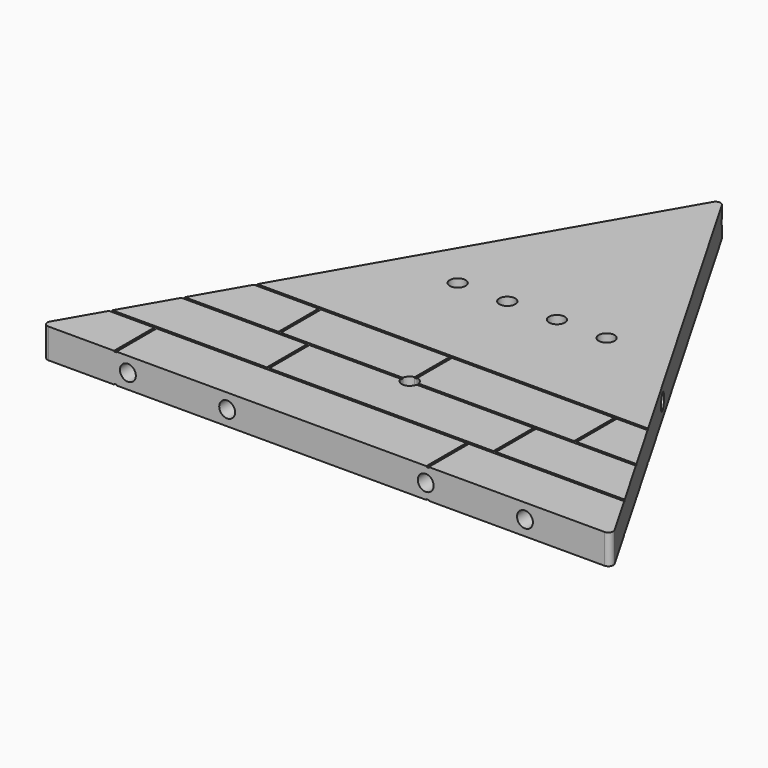
from build123d import *

# Parameters (mm, degrees)
F3_DEPTH       = 6
F4_W           = 32.6863850343
F4_H           = 10.1006624426
F4_W_2         = 25.8918322674
F5_DEPTH       = 0.15
F6_W           = 25.8918322674
F6_H           = 10.1006624426
F6_W_2         = 45.1567518413
F6_W_3         = 32.6863850343
F7_DEPTH       = 0.15
F8_R           = 1.6
F9_DEPTH       = 5
F11_R          = 1.05
F12_DEPTH      = 5
F12_DEPTH_BACK = 0.501
F13_R          = 1.6
F14_DEPTH      = 5
F15_R          = 1.6
F16_DEPTH      = 5
F17_R          = 1.6
F18_DEPTH      = 5


with BuildPart() as f3:
    # F2 (on Top) → F3 (new body)
    with BuildSketch(Plane.XY):
        with BuildLine():
            ThreePointArc((0.8660254038, 98.5), (0, 99), (-0.8660254038, 98.5))
            Line((-0.8660254038, 98.5), (-56.8690015152, 1.5))
            ThreePointArc((-56.8690015152, 1.5), (-56.8690015152, 0.5), (-56.0029761114, 0))
            Line((-56.0029761114, 0), (56.0029761114, 0))
            ThreePointArc((56.0029761114, 0), (56.8690015152, 0.5), (56.8690015152, 1.5))
            Line((56.8690015152, 1.5), (0.8660254038, 98.5))
        make_face()
    extrude(amount=F3_DEPTH)

    # F4 (on face) → F5 (cut)
    with BuildSketch(Plane.XY.offset(6)):
        Polygon((39.6628161091, 31.3019873277), (39.3741409745, 31.8019873277), (0, 31.8019873277), (0, 20.7013248852), (25.1688986466, 20.7013248852), (25.1688986466, 10.6006624426), (0, 10.6006624426), (0, 10.1006624426), (20.1229155064, 10.1006624426), (20.1229155064, 0), (20.6229155064, 0), (20.6229155064, 10.1006624426), (51.9034067387, 10.1006624426), (51.6147316042, 10.6006624426), (25.6688986466, 10.6006624426), (25.6688986466, 20.7013248852), (45.7831114239, 20.7013248852), (45.4944362893, 21.2013248852), (33.4497465572, 21.2013248852), (33.4497465572, 31.3019873277), align=None)
        with Locations((16.60655404, 26.2516561065)):
            Rectangle(F4_W, F4_H, mode=Mode.SUBTRACT)
        Polygon((0, 20.7013248852), (0, 31.8019873277), (-39.3741409745, 31.8019873277), (-39.6628161091, 31.3019873277), (-26.6284707446, 31.3019873277), (-26.6284707446, 21.2013248852), (-45.4944362893, 21.2013248852), (-45.7831114239, 20.7013248852), (-20.4878531947, 20.7013248852), (-20.4878531947, 10.6006624426), (-51.6147316042, 10.6006624426), (-51.9034067387, 10.1006624426), (-42.7899323404, 10.1006624426), (-42.7899323404, 0), (-42.2899323404, 0), (-42.2899323404, 10.1006624426), (0, 10.1006624426), (0, 10.6006624426), (-19.9878531947, 10.6006624426), (-19.9878531947, 20.7013248852), align=None)
        with Locations((-13.1825546109, 26.2516561065)):
            Rectangle(F4_W_2, F4_H, mode=Mode.SUBTRACT)
    extrude(amount=-F5_DEPTH, mode=Mode.SUBTRACT)

    # F6 (on face) → F7 (cut)
    with BuildSketch(Plane.XY):
        Polygon((-51.9034067387, 10.1006624426), (-42.7899323404, 10.1006624426), (-42.7899323404, 0), (-42.2899323404, 0), (-42.2899323404, 10.1006624426), (20.1229155064, 10.1006624426), (20.1229155064, 0), (20.6229155064, 0), (20.6229155064, 10.1006624426), (51.9034067387, 10.1006624426), (51.6147316042, 10.6006624426), (25.6688986466, 10.6006624426), (25.6688986466, 20.7013248852), (45.7831114239, 20.7013248852), (45.4944362893, 21.2013248852), (33.4497465572, 21.2013248852), (33.4497465572, 31.3019873277), (39.6628161091, 31.3019873277), (39.3741409745, 31.8019873277), (-39.3741409745, 31.8019873277), (-39.6628161091, 31.3019873277), (-26.6284707446, 31.3019873277), (-26.6284707446, 21.2013248852), (-45.4944362893, 21.2013248852), (-45.7831114239, 20.7013248852), (-20.4878531947, 20.7013248852), (-20.4878531947, 10.6006624426), (-51.6147316042, 10.6006624426), align=None)
        with Locations((-13.1825546109, 26.2516561065)):
            Rectangle(F6_W, F6_H, mode=Mode.SUBTRACT)
        with Locations((2.5905227259, 15.6509936639)):
            Rectangle(F6_W_2, F6_H, mode=Mode.SUBTRACT)
        with Locations((16.60655404, 26.2516561065)):
            Rectangle(F6_W_3, F6_H, mode=Mode.SUBTRACT)
    extrude(amount=F7_DEPTH, mode=Mode.SUBTRACT)

    # F8 (on face) → F9 (cut)
    with BuildSketch(Plane.XY.offset(6)):
        with BuildLine():
            ThreePointArc((1.5937095858, 20.7013248852), (1.6084409724, 20.8259392813), (1.6133615229, 20.9513248852))
            ThreePointArc((1.6133615229, 20.9513248852), (1.6084409724, 21.076710489), (1.5937095858, 21.2013248852))
            ThreePointArc((1.5937095858, 21.2013248852), (1.1447323728, 22.0826957351), (0.2633615229, 22.5316729481))
            ThreePointArc((0.2633615229, 22.5316729481), (0.0133615229, 22.5513248852), (-0.2366384771, 22.5316729481))
            ThreePointArc((-0.2366384771, 22.5316729481), (-1.118009327, 22.0826957351), (-1.5669865401, 21.2013248852))
            ThreePointArc((-1.5669865401, 21.2013248852), (-1.5866384771, 20.9513248852), (-1.5669865401, 20.7013248852))
            ThreePointArc((-1.5669865401, 20.7013248852), (0.0133615229, 19.3513248852), (1.5937095858, 20.7013248852))
        make_face()
        with Locations((5, 51.8019873277)):
            Circle(F8_R)
        with Locations((-5, 51.8019873277)):
            Circle(F8_R)
        with Locations((15, 51.8019873277)):
            Circle(F8_R)
        with Locations((-15, 51.8019873277)):
            Circle(F8_R)
    extrude(amount=-F9_DEPTH, mode=Mode.SUBTRACT)

    # F11 (on 3pt) → F12 (cut, two sides)
    with BuildSketch(Plane.XZ.offset(-98.5)) as f12_sk:
        with Locations((0, 3)):
            Circle(F11_R)
    extrude(amount=F12_DEPTH, mode=Mode.SUBTRACT)
    extrude(f12_sk.sketch, amount=-F12_DEPTH_BACK, mode=Mode.SUBTRACT)

    # F13 (on face) → F14 (cut)
    with BuildSketch(Plane.XZ):
        with Locations((-40, 3)):
            Circle(F13_R)
        with Locations((-20, 3)):
            Circle(F13_R)
        with Locations((20, 3)):
            Circle(F13_R)
        with Locations((40, 3)):
            Circle(F13_R)
    extrude(amount=-F14_DEPTH, mode=Mode.SUBTRACT)

    # F15 (on face) → F16 (cut)
    with BuildSketch(Plane(origin=(43.3012701892, 25, 0), x_dir=(-0.5, 0.8660254038, 0), z_dir=(0.8660254038, 0.5, 0))):
        with Locations((22.8645373481, 3)):
            Circle(F15_R)
    extrude(amount=-F16_DEPTH, mode=Mode.SUBTRACT)

    # F17 (on face) → F18 (cut)
    with BuildSketch(Plane(origin=(-43.3012701892, 25, 0), x_dir=(-0.5, -0.8660254038, 0), z_dir=(-0.8660254038, 0.5, 0))):
        with Locations((-22.8645373481, 3)):
            Circle(F17_R)
    extrude(amount=-F18_DEPTH, mode=Mode.SUBTRACT)


solid = f3.part
